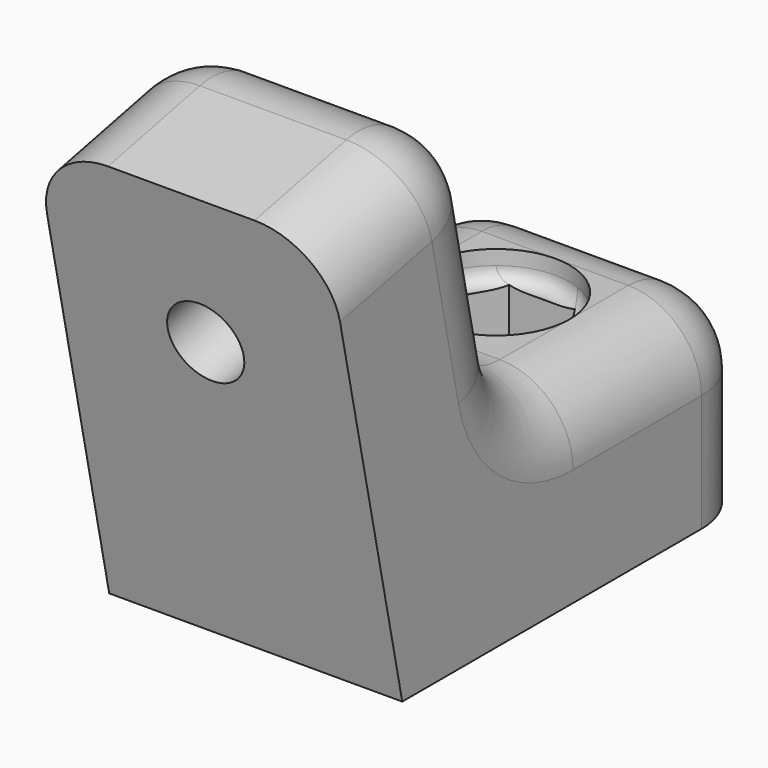
from build123d import *

# Parameters (mm, degrees)
F4_DEPTH  = 20
F5_R      = 2.6
F6_DEPTH  = 19.2092638861
F7_DEPTH  = 8
F5_R_2    = 5
F8_DEPTH  = 2
F9_R      = 2.6
F10_DEPTH = 13.001
F11_DEPTH = 8
F9_R_2    = 5
F12_DEPTH = 2
F14_R     = 5
F15_R     = 4.99999


# Not quite as in the source:
# - a fillet or chamfer that OpenCascade refuses, or shapes differently, is made with other operations: its cross-section is extruded or revolved along the edge and cut away or added
# - a fillet or chamfer is up to 0.001 mm smaller than in the source, because OpenCascade refuses the exact size


with BuildPart() as f4:
    # F3 (on Right) → F4 (new body)
    with BuildSketch(Plane.YZ):
        Polygon((-6.3469601944, 29.860100034), (0, 0), (30.5271924315, 0), (30.5271924315, 13), (10.5271924315, 13), (6.3689586152, 32.5629520147), align=None)
    extrude(amount=F4_DEPTH)

    # F5 (on face) → F6 (cut, through all)
    with BuildSketch(Plane(origin=(0, 12.7159188095, 2.7028519806), x_dir=(-1, 0, 0), z_dir=(0, 0.9781476007, 0.2079116908))):
        with Locations((-10, 20.5271924315)):
            Circle(F5_R)
    extrude(amount=-F6_DEPTH, mode=Mode.SUBTRACT)

    # F5 (on face) → F7 (cut)
    with BuildSketch(Plane(origin=(0, 12.7159188095, 2.7028519806), x_dir=(-1, 0, 0), z_dir=(0, 0.9781476007, 0.2079116908))):
        Polygon((-7.75, 24.4243067486), (-12.25, 24.4243067486), (-14.5, 20.5271924315), (-12.25, 16.6300781145), (-7.75, 16.6300781145), (-5.5, 20.5271924315), align=None)
        with Locations((-10, 20.5271924315)):
            Circle(F5_R, mode=Mode.SUBTRACT)
    extrude(amount=-F7_DEPTH, mode=Mode.SUBTRACT)

    # F5 (on face) → F8 (cut)
    with BuildSketch(Plane(origin=(0, 12.7159188095, 2.7028519806), x_dir=(-1, 0, 0), z_dir=(0, 0.9781476007, 0.2079116908))):
        with Locations((-10, 20.5271924315)):
            Circle(F5_R_2)
        Polygon((-14.5, 20.5271924315), (-12.25, 24.4243067486), (-7.75, 24.4243067486), (-5.5, 20.5271924315), (-7.75, 16.6300781145), (-12.25, 16.6300781145), align=None, mode=Mode.SUBTRACT)
    extrude(amount=-F8_DEPTH, mode=Mode.SUBTRACT)

    # F9 (on face) → F10 (cut, through all)
    with BuildSketch(Plane.XY.offset(13)):
        with Locations((10, 20.5271924315)):
            Circle(F9_R)
    extrude(amount=-F10_DEPTH, mode=Mode.SUBTRACT)

    # F9 (on face) → F11 (cut)
    with BuildSketch(Plane.XY.offset(13)):
        Polygon((12.25, 24.4243067486), (7.75, 24.4243067486), (5.5, 20.5271924315), (7.75, 16.6300781145), (12.25, 16.6300781145), (14.5, 20.5271924315), align=None)
        with Locations((10, 20.5271924315)):
            Circle(F9_R, mode=Mode.SUBTRACT)
    extrude(amount=-F11_DEPTH, mode=Mode.SUBTRACT)

    # F9 (on face) → F12 (cut)
    with BuildSketch(Plane.XY.offset(13)):
        with Locations((10, 20.5271924315)):
            Circle(F9_R_2)
        Polygon((5.5, 20.5271924315), (7.75, 24.4243067486), (12.25, 24.4243067486), (14.5, 20.5271924315), (12.25, 16.6300781145), (7.75, 16.6300781145), align=None, mode=Mode.SUBTRACT)
    extrude(amount=-F12_DEPTH, mode=Mode.SUBTRACT)

    # F13: fillet of radius 1 on 2 edges, made by hand


with BuildPart() as f13_tool2:
    # F13_s3 → F13_t4 (revolve)
    with BuildSketch(Plane(origin=(0, -4.2678432862, 20.0786240267), x_dir=(1, 0, 0), z_dir=(0, 0.2079116908, -0.9781476007))):
        with BuildLine():
            ThreePointArc((5, -12), (5.2928932188, -11.2928932188), (6, -11))
            Line((6, -11), (5, -11))
            Line((5, -11), (5, -12))
        make_face()
    revolve(axis=Axis((10, 6.4917803219, 22.3656526257), (0, 0.9781476007, 0.2079116908)))

    split(bisect_by=Plane(origin=(-4.763535057, -0.5718046051, 2.6901291617), x_dir=(0.1191822875, -0.9928723898, 0), z_dir=(-0.8660254038, -0.1039558454, 0.4890738004)), keep=Keep.TOP)


with BuildPart() as f4_1:
    add(f4.part)

    # F13_t1: union F13_tool2
    add(f13_tool2.part)


with BuildPart() as f13_tool7:
    # F13_s8 → F13_t9 (revolve)
    with BuildSketch(Plane(origin=(0, -4.2678432862, 20.0786240267), x_dir=(1, 0, 0), z_dir=(0, 0.2079116908, -0.9781476007))):
        with BuildLine():
            ThreePointArc((5, -12), (5.2928932188, -11.2928932188), (6, -11))
            Line((6, -11), (5, -11))
            Line((5, -11), (5, -12))
        make_face()
    revolve(axis=Axis((10, 6.4917803219, 22.3656526257), (0, 0.9781476007, 0.2079116908)))

    split(bisect_by=Plane(origin=(13.013535057, -1.562117038, 7.3491828516), x_dir=(-0.1191822875, -0.9928723898, 0), z_dir=(-0.8660254038, 0.1039558454, -0.4890738004)), keep=Keep.TOP)


with BuildPart() as f4_2:
    add(f4_1.part)

    # F13_t6: union F13_tool7
    add(f13_tool7.part)


with BuildPart() as f13_tool12:
    # F13_s13 → F13_t14 (revolve)
    with BuildSketch(Plane(origin=(0, -4.2678432862, 20.0786240267), x_dir=(1, 0, 0), z_dir=(0, 0.2079116908, -0.9781476007))):
        with BuildLine():
            ThreePointArc((5, -12), (5.2928932188, -11.2928932188), (6, -11))
            Line((6, -11), (5, -11))
            Line((5, -11), (5, -12))
        make_face()
    revolve(axis=Axis((10, 6.4917803219, 22.3656526257), (0, 0.9781476007, 0.2079116908)))

    split(bisect_by=Plane(origin=(0, -5.0780989131, 23.8905770457), x_dir=(1, 0, 0), z_dir=(0, -0.2079116908, 0.9781476007)), keep=Keep.TOP)


with BuildPart() as f4_3:
    add(f4_2.part)

    # F13_t11: union F13_tool12
    add(f13_tool12.part)


with BuildPart() as f13_tool17:
    # F13_s18 → F13_t19 (revolve)
    with BuildSketch(Plane(origin=(0, -4.2678432862, 20.0786240267), x_dir=(1, 0, 0), z_dir=(0, 0.2079116908, -0.9781476007))):
        with BuildLine():
            ThreePointArc((5, -12), (5.2928932188, -11.2928932188), (6, -11))
            Line((6, -11), (5, -11))
            Line((5, -11), (5, -12))
        make_face()
    revolve(axis=Axis((10, 6.4917803219, 22.3656526257), (0, 0.9781476007, 0.2079116908)))

    split(bisect_by=Plane(origin=(0, -3.4575876592, 16.2666710077), x_dir=(1, 0, 0), z_dir=(0, 0.2079116908, -0.9781476007)), keep=Keep.TOP)


with BuildPart() as f4_4:
    add(f4_3.part)

    # F13_t16: union F13_tool17
    add(f13_tool17.part)


with BuildPart() as f13_tool22:
    # F13_s23 → F13_t24 (revolve)
    with BuildSketch(Plane(origin=(0, -4.2678432862, 20.0786240267), x_dir=(1, 0, 0), z_dir=(0, 0.2079116908, -0.9781476007))):
        with BuildLine():
            ThreePointArc((5, -12), (5.2928932188, -11.2928932188), (6, -11))
            Line((6, -11), (5, -11))
            Line((5, -11), (5, -12))
        make_face()
    revolve(axis=Axis((10, 6.4917803219, 22.3656526257), (0, 0.9781476007, 0.2079116908)))

    split(bisect_by=Plane(origin=(19.763535057, -2.372372665, 11.1611358706), x_dir=(0.1191822875, 0.9928723898, 0), z_dir=(0.8660254038, -0.1039558454, 0.4890738004)), keep=Keep.TOP)


with BuildPart() as f4_5:
    add(f4_4.part)

    # F13_t21: union F13_tool22
    add(f13_tool22.part)


with BuildPart() as f13_tool27:
    # F13_s28 → F13_t29 (revolve)
    with BuildSketch(Plane(origin=(0, -4.2678432862, 20.0786240267), x_dir=(1, 0, 0), z_dir=(0, 0.2079116908, -0.9781476007))):
        with BuildLine():
            ThreePointArc((5, -12), (5.2928932188, -11.2928932188), (6, -11))
            Line((6, -11), (5, -11))
            Line((5, -11), (5, -12))
        make_face()
    revolve(axis=Axis((10, 6.4917803219, 22.3656526257), (0, 0.9781476007, 0.2079116908)))

    split(bisect_by=Plane(origin=(1.986464943, 0.2384510219, -1.1218238572), x_dir=(-0.1191822875, 0.9928723898, 0), z_dir=(0.8660254038, 0.1039558454, -0.4890738004)), keep=Keep.TOP)


with BuildPart() as f4_6:
    add(f4_5.part)

    # F13_t26: union F13_tool27
    add(f13_tool27.part)


with BuildPart() as f13_tool32:
    # F13_s33 → F13_t34 (revolve)
    with BuildSketch(Plane.XZ.offset(-20.5271924315)):
        with BuildLine():
            ThreePointArc((15, 12), (14.7071067812, 11.2928932188), (14, 11))
            Line((14, 11), (15, 11))
            Line((15, 11), (15, 12))
        make_face()
    revolve(axis=Axis((10, 20.5271924315, 11), (0, 0, 1)))

    split(bisect_by=Plane(origin=(19.763535057, 11.4104822853, 0), x_dir=(0, 0, 1), z_dir=(0.8660254038, 0.5, 0)), keep=Keep.TOP)


with BuildPart() as f4_7:
    add(f4_6.part)

    # F13_t31: union F13_tool32
    add(f13_tool32.part)


with BuildPart() as f13_tool37:
    # F13_s38 → F13_t39 (revolve)
    with BuildSketch(Plane.XZ.offset(-20.5271924315)):
        with BuildLine():
            ThreePointArc((15, 12), (14.7071067812, 11.2928932188), (14, 11))
            Line((14, 11), (15, 11))
            Line((15, 11), (15, 12))
        make_face()
    revolve(axis=Axis((10, 20.5271924315, 11), (0, 0, 1)))

    split(bisect_by=Plane(origin=(1.986464943, -1.1468860696, 0), x_dir=(0, 0, 1), z_dir=(0.8660254038, -0.5, 0)), keep=Keep.TOP)


with BuildPart() as f4_8:
    add(f4_7.part)

    # F13_t36: union F13_tool37
    add(f13_tool37.part)


with BuildPart() as f13_tool42:
    # F13_s43 → F13_t44 (revolve)
    with BuildSketch(Plane.XZ.offset(-20.5271924315)):
        with BuildLine():
            ThreePointArc((15, 12), (14.7071067812, 11.2928932188), (14, 11))
            Line((14, 11), (15, 11))
            Line((15, 11), (15, 12))
        make_face()
    revolve(axis=Axis((10, 20.5271924315, 11), (0, 0, 1)))

    split(bisect_by=Plane.XZ.offset(-24.4243067486), keep=Keep.BOTTOM)


with BuildPart() as f4_9:
    add(f4_8.part)

    # F13_t41: union F13_tool42
    add(f13_tool42.part)


with BuildPart() as f13_tool47:
    # F13_s48 → F13_t49 (revolve)
    with BuildSketch(Plane.XZ.offset(-20.5271924315)):
        with BuildLine():
            ThreePointArc((15, 12), (14.7071067812, 11.2928932188), (14, 11))
            Line((14, 11), (15, 11))
            Line((15, 11), (15, 12))
        make_face()
    revolve(axis=Axis((10, 20.5271924315, 11), (0, 0, 1)))

    split(bisect_by=Plane.XZ.offset(-16.6300781145), keep=Keep.TOP)


with BuildPart() as f4_10:
    add(f4_9.part)

    # F13_t46: union F13_tool47
    add(f13_tool47.part)


with BuildPart() as f13_tool52:
    # F13_s53 → F13_t54 (revolve)
    with BuildSketch(Plane.XZ.offset(-20.5271924315)):
        with BuildLine():
            ThreePointArc((15, 12), (14.7071067812, 11.2928932188), (14, 11))
            Line((14, 11), (15, 11))
            Line((15, 11), (15, 12))
        make_face()
    revolve(axis=Axis((10, 20.5271924315, 11), (0, 0, 1)))

    split(bisect_by=Plane(origin=(-4.763535057, 2.7502282475, 0), x_dir=(0, 0, 1), z_dir=(-0.8660254038, 0.5, 0)), keep=Keep.TOP)


with BuildPart() as f4_11:
    add(f4_10.part)

    # F13_t51: union F13_tool52
    add(f13_tool52.part)


with BuildPart() as f13_tool57:
    # F13_s58 → F13_t59 (revolve)
    with BuildSketch(Plane.XZ.offset(-20.5271924315)):
        with BuildLine():
            ThreePointArc((15, 12), (14.7071067812, 11.2928932188), (14, 11))
            Line((14, 11), (15, 11))
            Line((15, 11), (15, 12))
        make_face()
    revolve(axis=Axis((10, 20.5271924315, 11), (0, 0, 1)))

    split(bisect_by=Plane(origin=(13.013535057, 7.5133679683, 0), x_dir=(0, 0, 1), z_dir=(-0.8660254038, -0.5, 0)), keep=Keep.TOP)


with BuildPart() as f4_12:
    add(f4_11.part)

    # F13_t56: union F13_tool57
    add(f13_tool57.part)

    # F14
    f14_edges = [f4_12.edges().sort_by_distance(p)[0] for p in [
        (10, 10.527192, 13),
    ]]
    fillet(f14_edges, radius=F14_R)

    # F15 (radius 5 in the source; OpenCascade refuses exactly that, so slightly less here)
    f15_edges = [f4_12.edges().sort_by_distance(p)[0] for p in [
        (20, 0.010999, 31.211526),
        (20, 8.027167, 24.761697),
        (20, 30.527192, 6.5),
        (0, 30.527192, 6.5),
        (0, 22.551653, 13),
        (0, 0.010999, 31.211526),
        (10, 30.527192, 13),
        (10, 6.368959, 32.562952),
        (0, 11.429511, 14.11427),
        (20, 11.429511, 14.11427),
    ]]
    fillet(f15_edges, radius=F15_R)


solid = f4_12.part
